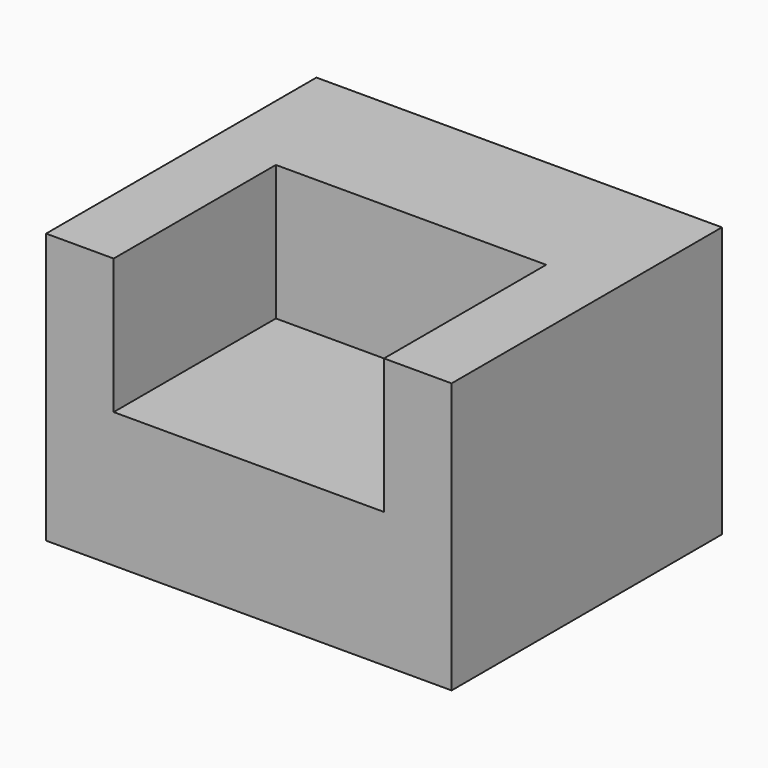
from build123d import *

# Parameters (mm, degrees)
F1_DEPTH = 76.2
F2_W     = 101.6
F2_H     = 50.8
F3_DEPTH = 50.8


with BuildPart() as f1:
    # F0 (on Front) → F1 (new body)
    with BuildSketch(Plane.XZ):
        Polygon((-68.4001594782, 53.9017294705), (-68.4001594782, -47.6982705295), (83.9998405218, -47.6982705295), (83.9998405218, 53.9017294705), (58.5998405218, 53.9017294705), (58.5998405218, 3.1017294705), (-43.0001594782, 3.1017294705), (-43.0001594782, 53.9017294705), align=None)
    extrude(amount=F1_DEPTH)

    # F2 (on face) → F3 (join)
    with BuildSketch(Plane(origin=(0, 0, 0), x_dir=(-1, 0, 0), z_dir=(0, 1, 0))):
        with Locations((-7.7998405218, 28.5017294705)):
            Rectangle(F2_W, F2_H)
        Polygon((-58.5998405218, 53.9017294705), (-83.9998405218, 53.9017294705), (-83.9998405218, -47.6982705295), (68.4001594782, -47.6982705295), (68.4001594782, 53.9017294705), (43.0001594782, 53.9017294705), (43.0001594782, 3.1017294705), (-58.5998405218, 3.1017294705), align=None)
    extrude(amount=F3_DEPTH)


solid = f1.part
